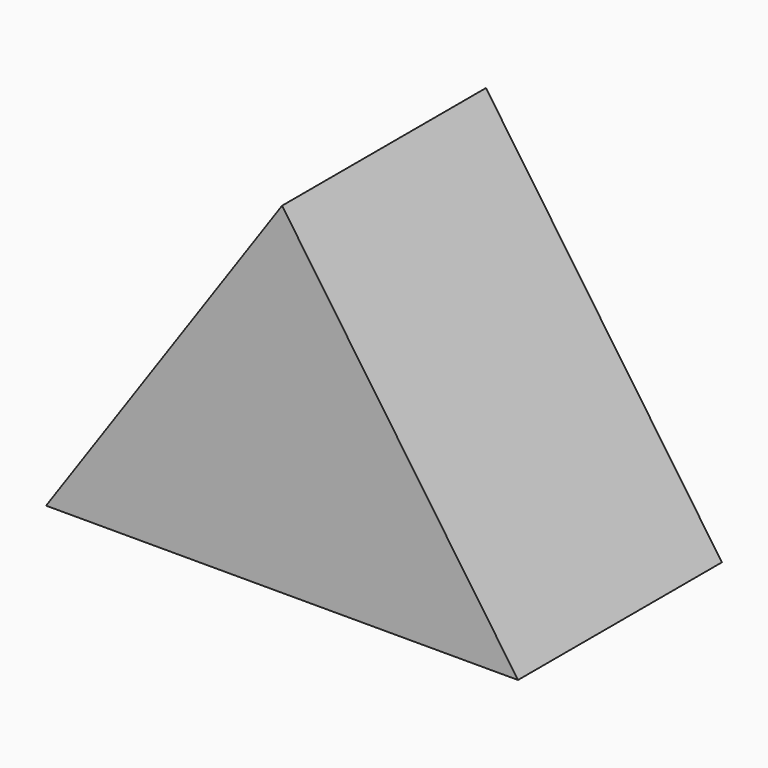
from build123d import *

# Parameters (mm, degrees)
F1_DEPTH = 85344


# Not quite as in the source:
# - a feature names something its author has since deleted; it is built from what else it names


with BuildPart() as f1:
    # F0 (on Front) → F1 (new body)
    with BuildSketch(Plane.XZ):
        Polygon((79012.0669388851, 114123.5151276526), (0, 0), (158024.1338777702, 0), align=None)
    extrude(amount=F1_DEPTH)


solid = f1.part
